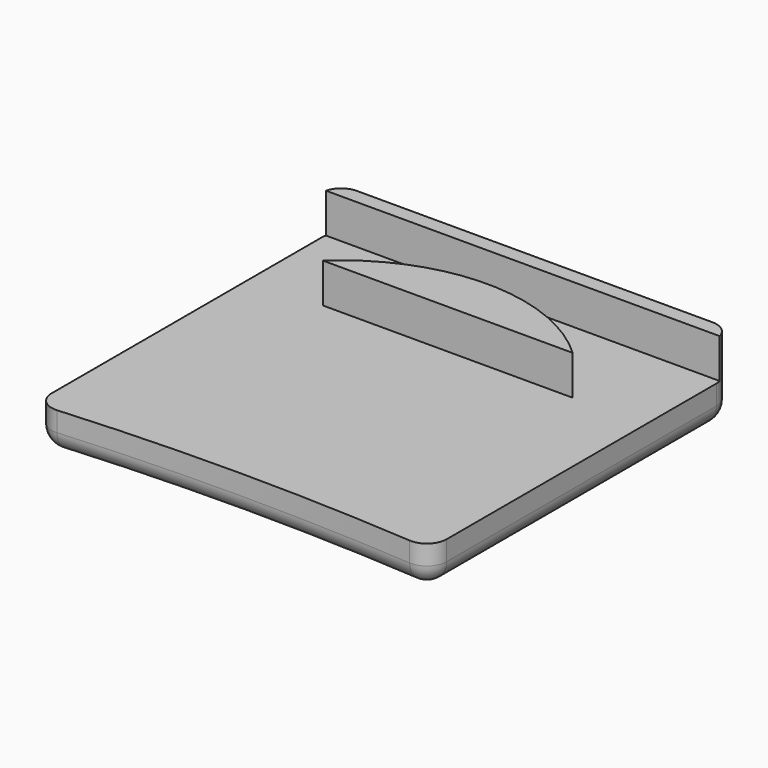
from build123d import *

# Parameters (mm, degrees)
F0_W     = 20
F0_H     = 22
F1_DEPTH = 2
F2_R     = 9.25
F4_DEPTH = 2
F3_W     = 20
F3_H     = 18
F5_DEPTH = 2
F6_W     = 20
F6_H     = 0.75
F7_DEPTH = 2
F8_R     = 125
F9_DEPTH = 2
F10_R    = 1


with BuildPart() as f1:
    # F0 (on Top) → F1 (new body)
    with BuildSketch(Plane.XY):
        Rectangle(F0_W, F0_H)
    extrude(amount=F1_DEPTH)

    # F2 (on face) → F4 (join)
    with BuildSketch(Plane.XY.offset(2)):
        with Locations((0, -1.25)):
            Circle(F2_R)
    extrude(amount=F4_DEPTH)

    # F3 (on face) → F5 (cut)
    with BuildSketch(Plane.XY.offset(2)):
        with Locations((0, -3.5)):
            Rectangle(F3_W, F3_H)
    extrude(amount=F5_DEPTH, mode=Mode.SUBTRACT)

    # F6 (on face) → F7 (join)
    with BuildSketch(Plane.XY.offset(2)):
        with Locations((0, 10.625)):
            Rectangle(F6_W, F6_H)
    extrude(amount=F7_DEPTH)

    # F8 (on Top) → F9 (cut)
    with BuildSketch(Plane.XY):
        with Locations((0, -132.75)):
            Circle(F8_R)
    extrude(amount=F9_DEPTH, mode=Mode.SUBTRACT)

    # F10
    f10_edges = [f1.edges().sort_by_distance(p)[0] for p in [
        (10, -8.150642, 1),
        (-10, -8.150642, 1),
        (10, 11, 2),
        (-10, 11, 2),
        (0, 11, 0),
        (-10, 1.424679, 0),
        (0, -7.75, 0),
        (10, 1.424679, 0),
    ]]
    fillet(f10_edges, radius=F10_R)


solid = f1.part
